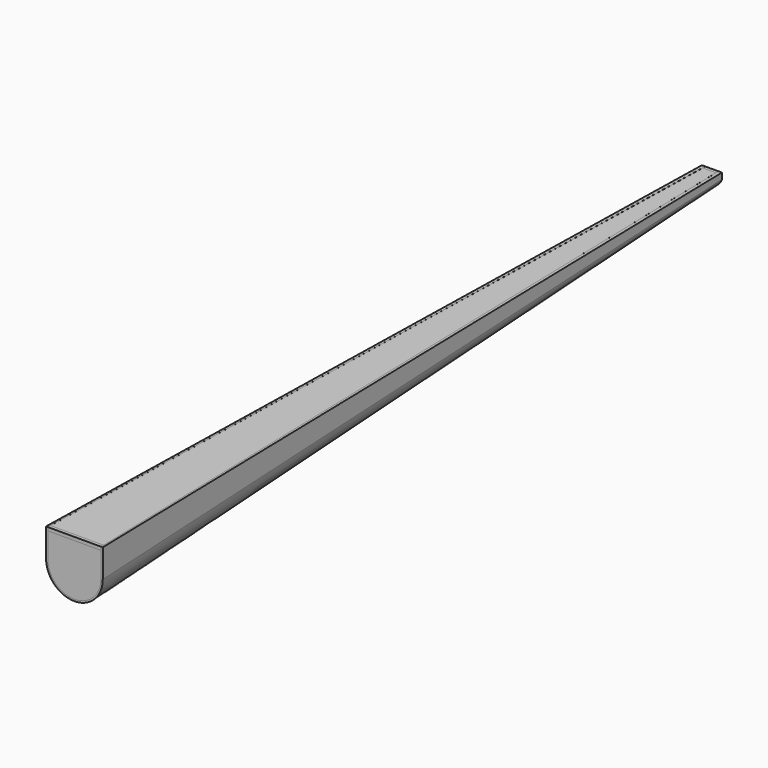
from build123d import *

# Parameters (mm, degrees)
F1_DEPTH  = 3.175
F0_W      = 1.6933333333
F0_H      = 3.2089926077
F3_W      = 3.175
F3_H      = 3.2089926077
F7_DEPTH  = 3.175
F8_DEPTH  = 3.175
F9_DEPTH  = 3.175
F9_FACE_W = 50.8
F9_FACE_H = 3.175
F8_FACE_W = 12.7
F8_FACE_H = 3.175


with BuildPart() as f1:
    # F0 (on Front) → F1 (new body)
    with BuildSketch(Plane.XZ):
        with BuildLine():
            Line((25.4, -13.5466666667), (25.4, 10.337674059))
            Line((25.4, 10.337674059), (-25.4, 10.337674059))
            Line((-25.4, 10.337674059), (-25.4, -13.5466666667))
            ThreePointArc((-25.4, -13.5466666667), (0, -38.9466666667), (25.4, -13.5466666667))
        make_face()
    extrude(amount=-F1_DEPTH)


with BuildPart() as f4:
    # F0 (on Front) → F4 section 0
    with BuildSketch(Plane.XZ):
        with BuildLine():
            ThreePointArc((-27.0933333333, -13.5466666667), (0, -40.64), (27.0933333333, -13.5466666667))
            Line((27.0933333333, -13.5466666667), (27.0933333333, 10.337674059))
            Line((27.0933333333, 10.337674059), (25.4, 10.337674059))
            Line((25.4, 10.337674059), (25.4, -13.5466666667))
            ThreePointArc((25.4, -13.5466666667), (0, -38.9466666667), (-25.4, -13.5466666667))
            Line((-25.4, -13.5466666667), (-25.4, 10.337674059))
            Line((-25.4, 10.337674059), (-27.0933333333, 10.337674059))
            Line((-27.0933333333, 10.337674059), (-27.0933333333, -13.5466666667))
        make_face()
    # F3 (on offset) → F4 section 1
    with BuildSketch(Plane.XZ.offset(-762)):
        with BuildLine():
            Line((-6.35, 10.337674059), (-9.525, 10.337674059))
            Line((-9.525, 10.337674059), (-9.525, 7.797674059))
            ThreePointArc((-9.525, 7.797674059), (0, 0.4798231268), (9.525, 7.797674059))
            Line((9.525, 7.797674059), (9.525, 10.337674059))
            Line((9.525, 10.337674059), (6.35, 10.337674059))
            Line((6.35, 10.337674059), (6.35, 7.797674059))
            ThreePointArc((6.35, 7.797674059), (0, 3.4985147539), (-6.35, 7.797674059))
            Line((-6.35, 7.797674059), (-6.35, 10.337674059))
        make_face()
    loft()

    # F0 (on Front) → F5 section 0
    with BuildSketch(Plane.XZ):
        with Locations((-26.2466666667, 11.9421703628)):
            Rectangle(F0_W, F0_H)
    # F3 (on offset) → F5 section 1
    with BuildSketch(Plane.XZ.offset(-762)):
        with Locations((-7.9375, 11.9421703628)):
            Rectangle(F3_W, F3_H)
    loft()

    # F0 (on Front) → F6 section 0
    with BuildSketch(Plane.XZ):
        with Locations((26.2466666667, 11.9421703628)):
            Rectangle(F0_W, F0_H)
    # F3 (on offset) → F6 section 1
    with BuildSketch(Plane.XZ.offset(-762)):
        with Locations((7.9375, 11.9421703628)):
            Rectangle(F3_W, F3_H)
    loft()


with BuildPart() as f7:
    # F3 (on offset) → F7 (new body)
    with BuildSketch(Plane.XZ.offset(-762)):
        with BuildLine():
            Line((6.35, 10.337674059), (-6.35, 10.337674059))
            Line((-6.35, 10.337674059), (-6.35, 7.797674059))
            ThreePointArc((-6.35, 7.797674059), (0, 3.4985147539), (6.35, 7.797674059))
            Line((6.35, 7.797674059), (6.35, 10.337674059))
        make_face()
    extrude(amount=F7_DEPTH)


with BuildPart() as f8:
    # F8 (new): a face of the model
    f8_faces = [f7.part.faces().sort_by_distance(p)[0] for p in [
        (0, 760.4125, 10.337674059),
    ]]
    extrude(f8_faces, amount=F8_DEPTH)


with BuildPart() as f9:
    # F9 (new): a face of the model
    f9_faces = [f1.part.faces().sort_by_distance(p)[0] for p in [
        (0, 1.5875, 10.337674059),
    ]]
    extrude(f9_faces, amount=F9_DEPTH)


with BuildPart() as f10:
    # F9_face (on face) → F10 section 0
    with BuildSketch(Plane(origin=(0, 3.175, 11.925174059), x_dir=(-1, 0, 0), z_dir=(0, 1, 0))):
        Rectangle(F9_FACE_W, F9_FACE_H)
    # F8_face (on face) → F10 section 1
    with BuildSketch(Plane(origin=(0, 758.825, 11.925174059), x_dir=(1, 0, 0), z_dir=(0, -1, 0))):
        Rectangle(F8_FACE_W, F8_FACE_H)
    loft()


solid = Compound([f1.part, f4.part, f7.part, f8.part, f9.part, f10.part])
